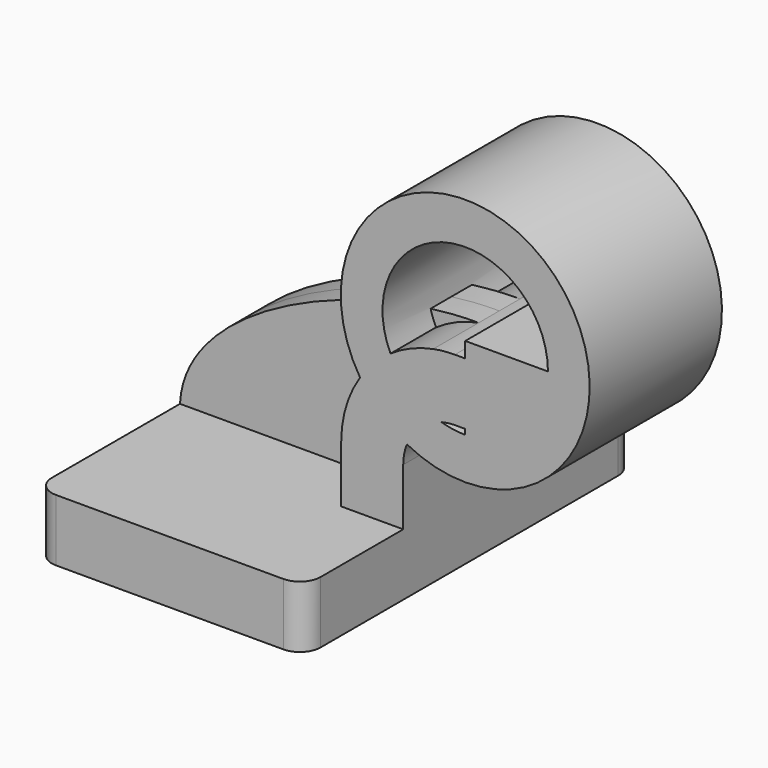
from build123d import *

# Parameters (mm, degrees)
F1_DEPTH  = 63.5
F2_DEPTH  = 25.4
F3_DEPTH  = 7.9375
F2_FACE_W = 50.8
F2_FACE_H = 28.575004
F5_R      = 6.35


# Not quite as in the source:
# - after a boolean that leaves OpenCascade's solid faulty, fix() repairs it


with BuildPart() as f1:
    # F0 (on Front) → F1 (new body, symmetric)
    with BuildSketch(Plane.XZ):
        Polygon((-41.275, 9.525), (-41.275, -9.525), (41.275, -9.525), (41.275, 9.525), (22.225, 9.525), align=None)
    extrude(amount=F1_DEPTH, both=True)

    # F0 (on Front) → F2 (join, symmetric)
    with BuildSketch(Plane.XZ):
        Polygon((-41.275, 9.525), (-41.275, -9.525), (41.275, -9.525), (41.275, 9.525), (22.225, 9.525), align=None)
        Polygon((85.727223, 42.8752), (60.325, 42.8752), (60.325, 38.1), (85.725, 38.1), align=None)
        Polygon((60.325, 66.675), (60.325, 61.9252), (85.73609, 61.9252), (85.738301, 66.675), align=None)
        Polygon((85.73609, 61.9252), (60.325, 61.9252), (60.325, 42.8752), (85.727223, 42.8752), align=None)
        with BuildLine():
            Line((22.225, 9.525), (41.275, 9.525))
            Line((41.275, 9.525), (41.275, 27.0002))
            ThreePointArc((41.275, 27.0002), (45.92468, 38.22552), (57.15, 42.8752))
            Line((57.15, 42.8752), (60.325, 42.8752))
            Line((60.325, 42.8752), (60.325, 61.9252))
            Line((60.325, 61.9252), (57.15, 61.9252))
            ThreePointArc((57.15, 61.9252), (53.796565, 61.763832), (50.474119, 61.281219))
            ThreePointArc((50.474119, 61.281219), (30.197164, 49.210563), (22.225, 27.0002))
            Line((22.225, 27.0002), (22.225, 9.525))
        make_face()
    extrude(amount=F2_DEPTH, both=True)

    # F0 (on Front) → F3 (join, symmetric)
    with BuildSketch(Plane.XZ):
        Polygon((-41.275, 9.525), (-41.275, -9.525), (41.275, -9.525), (41.275, 9.525), (22.225, 9.525), align=None)
        Polygon((85.727223, 42.8752), (60.325, 42.8752), (60.325, 38.1), (85.725, 38.1), align=None)
        Polygon((60.325, 66.675), (60.325, 61.9252), (85.73609, 61.9252), (85.738301, 66.675), align=None)
        with BuildLine():
            Line((22.225, 9.525), (41.275, 9.525))
            Line((41.275, 9.525), (41.275, 27.0002))
            ThreePointArc((41.275, 27.0002), (45.92468, 38.22552), (57.15, 42.8752))
            Line((57.15, 42.8752), (60.325, 42.8752))
            Line((60.325, 42.8752), (60.325, 61.9252))
            Line((60.325, 61.9252), (57.15, 61.9252))
            ThreePointArc((57.15, 61.9252), (53.796565, 61.763832), (50.474119, 61.281219))
            ThreePointArc((50.474119, 61.281219), (30.197164, 49.210563), (22.225, 27.0002))
            Line((22.225, 27.0002), (22.225, 9.525))
        make_face()
        Polygon((85.73609, 61.9252), (60.325, 61.9252), (60.325, 42.8752), (85.727223, 42.8752), align=None)
        with BuildLine():
            add(Edge.make_bspline(
                [(-41.275, 9.525), (-39.898027, 39.04913), (13.582303, 61.544828), (50.474119, 61.281219)],
                knots=[0, 0, 0, 0, 105.340434, 105.340434, 105.340434, 105.340434], degree=3))
            Line((-41.275, 9.525), (22.225, 9.525))
            Line((22.225, 9.525), (22.225, 27.0002))
            ThreePointArc((22.225, 27.0002), (30.197164, 49.210563), (50.474119, 61.281219))
        make_face()
    extrude(amount=F3_DEPTH, both=True)

    # F2_face (on face) → F4 (revolve)
    with BuildSketch(Plane(origin=(85.731651, 0, 52.3875), x_dir=(0, 1, 0), z_dir=(1, 0, -0.000465))):
        Rectangle(F2_FACE_W, F2_FACE_H)
    revolve(axis=Axis((60.325, 0, 66.675), (0, 1, 0)))

    add(f1.part.fix(), mode=Mode.REPLACE)

    # F5
    f5_edges = [f1.edges().sort_by_distance(p)[0] for p in [
        (-41.275, -63.5, 0),
        (-41.275, 63.5, 0),
        (41.275, -63.5, 0),
        (41.275, 63.5, 0),
    ]]
    fillet(f5_edges, radius=F5_R)


solid = f1.part
